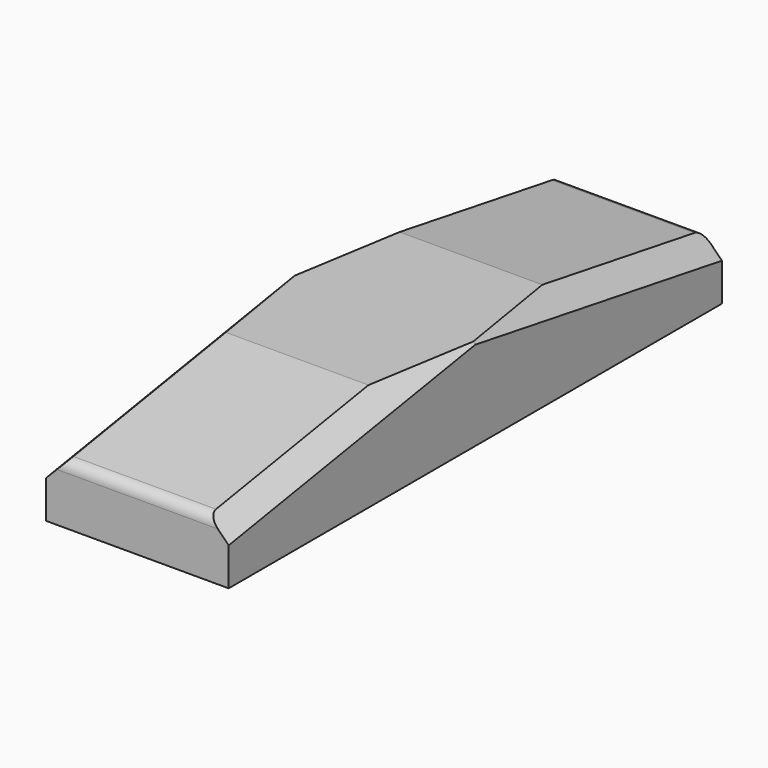
from build123d import *

# Parameters (mm, degrees)
F0_W        = 80
F0_H        = 279.619
F1_DEPTH    = 40
F2_SIZE2    = 90
F2_SIZE     = 15
F2_2_SIZE2  = 90
F2_2_SIZE   = 15
F3_SIZE     = 8
F4_T        = 2
F5_T1_DEPTH = 86.8350314591


# Not quite as in the source:
# - a fillet or chamfer that OpenCascade refuses, or shapes differently, is made with other operations: its cross-section is extruded or revolved along the edge and cut away or added


with BuildPart() as f1:
    # F0 (on Top) → F1 (new body)
    with BuildSketch(Plane.XY):
        Rectangle(F0_W, F0_H)
    extrude(amount=F1_DEPTH)

    # F2
    f2_edges = [f1.edges().sort_by_distance(p)[0] for p in [
        (0, 139.8095, 40),
    ]]
    f2_side = f1.faces().sort_by_distance((0, 139.8095, 20))[0]
    chamfer(f2_edges, length=F2_SIZE, length2=F2_SIZE2, reference=f2_side)

    # F2#2
    f2_2_edges = [f1.edges().sort_by_distance(p)[0] for p in [
        (0, -139.8095, 40),
    ]]
    f2_2_side = f1.faces().sort_by_distance((0, -139.8095, 20))[0]
    chamfer(f2_2_edges, length=F2_2_SIZE, length2=F2_2_SIZE2, reference=f2_2_side)

    # F3
    f3_edges = [f1.edges().sort_by_distance(p)[0] for p in [
        (-40, -94.8095, 32.5),
        (40, -94.8095, 32.5),
        (40, 94.8095, 32.5),
        (-40, 94.8095, 32.5),
    ]]
    chamfer(f3_edges, length=F3_SIZE)

    # F4
    f4_openings = [f1.faces().sort_by_distance(p)[0] for p in [
        (0, 0, 0),
    ]]
    offset(amount=F4_T, openings=f4_openings, kind=Kind.INTERSECTION)

    # F5: fillet of radius 5 on 2 edges, made by hand

    # F5_s2 → F5_t1 (cut)
    with BuildSketch(Plane.YZ.offset(-43.4175157295)):
        with BuildLine():
            ThreePointArc((-141.8095, 22.4586187349), (-140.6245999124, 25.6904932155), (-137.6314949365, 27.390588354))
            Line((-137.6314949365, 27.390588354), (-141.8095, 26.6942541768))
            Line((-141.8095, 26.6942541768), (-141.8095, 22.4586187349))
        make_face()
        with BuildLine():
            ThreePointArc((141.8095, 22.4586187349), (140.6245999124, 25.6904932155), (137.6314949365, 27.390588354))
            Line((137.6314949365, 27.390588354), (141.8095, 26.6942541768))
            Line((141.8095, 26.6942541768), (141.8095, 22.4586187349))
        make_face()
    extrude(amount=F5_T1_DEPTH, mode=Mode.SUBTRACT)


solid = f1.part
